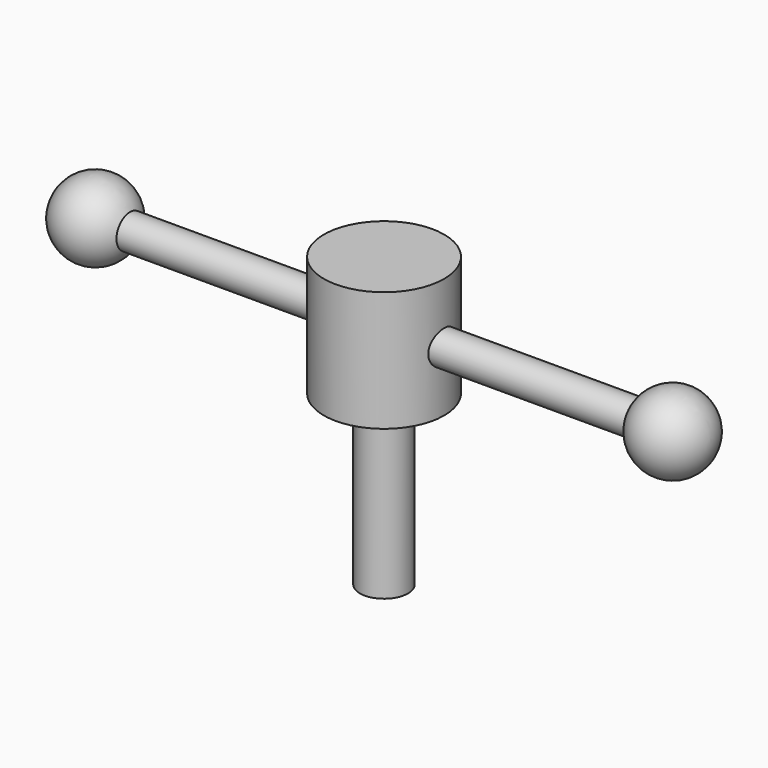
from build123d import *

# Parameters (mm, degrees)
F0_R          = 15.875
F0_R_2        = 6.35
F1_DEPTH      = 31.75
F2_DEPTH      = 44.45
F3_R          = 4.445
F4_DEPTH      = 76.2
F4_DEPTH_BACK = 76.2


with BuildPart() as f1:
    # F0 (on Top) → F1 (new body)
    with BuildSketch(Plane.XY):
        Circle(F0_R)
        Circle(F0_R_2, mode=Mode.SUBTRACT)
        Circle(F0_R_2)
    extrude(amount=F1_DEPTH)

    # F0 (on Top) → F2 (join)
    with BuildSketch(Plane.XY):
        Circle(F0_R_2)
    extrude(amount=-F2_DEPTH)

    # F3 (on Right) → F4 (join, two sides)
    with BuildSketch(Plane.YZ) as f4_sk:
        with Locations((0, 15.875)):
            Circle(F3_R)
    extrude(amount=-F4_DEPTH)
    extrude(f4_sk.sketch, amount=F4_DEPTH_BACK)

    # F5 (on Front) → F6 (revolve)
    with BuildSketch(Plane.XZ):
        with BuildLine():
            Line((-76.2, 15.875), (-66.04, 15.875))
            ThreePointArc((-66.04, 15.875), (-76.2, 26.035), (-86.36, 15.875))
            Line((-86.36, 15.875), (-76.2, 15.875))
        make_face()
    revolve(axis=Axis((-76.2, 0, 15.875), (-1, 0, 0)))

    # F5 (on Front) → F7 (revolve)
    with BuildSketch(Plane.XZ):
        with BuildLine():
            ThreePointArc((86.36, 15.875), (76.2, 26.035), (66.04, 15.875))
            Line((66.04, 15.875), (76.2, 15.875))
            Line((76.2, 15.875), (86.36, 15.875))
        make_face()
    revolve(axis=Axis((76.2, 0, 15.875), (1, 0, 0)))


solid = f1.part
